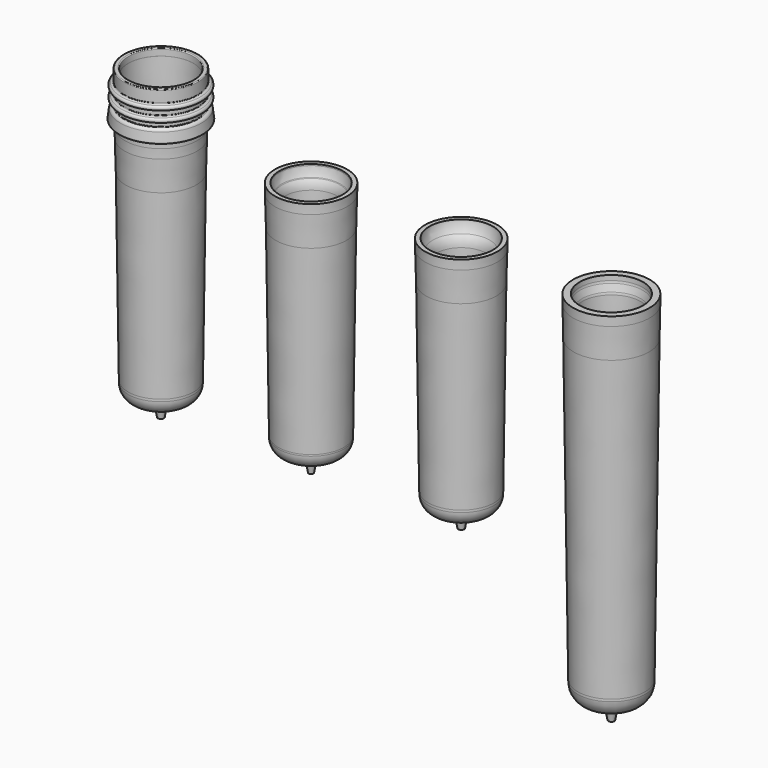
from build123d import *


# Not quite as in the source:
# - ends of sketch curves that miss each other by under 0.0002 mm in the source are joined


with BuildPart() as f2:
    # F1 (on Front) → F2 (revolve)
    with BuildSketch(Plane.XZ):
        with BuildLine():
            Line((-90.380559, 48.017019), (-90.3875184894, 48.4156921852))
            Line((-90.3875184894, 48.4156921852), (-91.848666, 48.396603))
            Line((-91.848666, 48.396603), (-91.808166, 45.296603))
            Line((-91.808166, 45.296603), (-91.546166, 35.296603))
            Line((-91.546166, 35.296603), (-90.748666, -25.603397))
            Line((-90.748666, -25.603397), (-90.724166, -25.603397))
            Line((-90.724166, -25.603397), (-90.714235, -26.362404))
            ThreePointArc((-90.714235, -26.362404), (-89.5797271662, -29.4689449214), (-86.7542219771, -31.1877308925))
            Line((-86.7542219771, -31.1877308925), (-84.798666, -31.603397))
            Line((-84.798666, -31.603397), (-82.5194, -31.603397))
            ThreePointArc((-82.5194, -31.603397), (-81.8766123734, -31.8373525711), (-81.5345922393, -32.4297488659))
            Line((-81.5345922393, -32.4297488659), (-80.798666, -36.603397))
            Line((-80.798666, -36.603397), (-79.797526, -36.603397))
            Line((-79.797526, -36.603397), (-79.797526, -30.103397))
            Line((-79.797526, -30.103397), (-83.797526, -30.103397))
            Line((-83.797526, -30.103397), (-86.010944, -29.163857))
            ThreePointArc((-86.010944, -29.163857), (-87.5492637787, -27.8929535328), (-88.1430844076, -25.9879599922))
            Line((-88.1430844076, -25.9879599922), (-88.945026, 35.296603))
            Line((-88.945026, 35.296603), (-89.032202, 42.663642))
            ThreePointArc((-89.032202, 42.663642), (-89.2114545385, 44.0499692845), (-89.7066271049, 45.3571949455))
            ThreePointArc((-89.7066271049, 45.3571949455), (-90.1976808008, 46.6480650102), (-90.380559, 48.017019))
        make_face()
    revolve(axis=Axis((-79.797526, 0, -33.353397), (0, 0, -1)))


with BuildPart() as f4:
    # F3 (on Front) → F4 (revolve)
    with BuildSketch(Plane.XZ):
        with BuildLine():
            Line((-90.3871852566, 48.396603), (-90.652526, 63.596603))
            Line((-90.652526, 63.596603), (-90.653015, 63.624612))
            Line((-90.653015, 63.624612), (-90.65259, 65.596538))
            ThreePointArc((-90.65259, 65.596538), (-90.7404349859, 65.8087120521), (-90.95259, 65.896603))
            Line((-90.95259, 65.896603), (-91.858666, 65.896603))
            ThreePointArc((-91.858666, 65.896603), (-92.0354426953, 65.8233796953), (-92.108666, 65.646603))
            Line((-92.108666, 65.646603), (-92.108666, 62.896603))
            Line((-92.108666, 62.896603), (-92.108666, 62.036644))
            ThreePointArc((-92.108666, 62.036644), (-92.1448355475, 61.9219287751), (-92.2402618282, 61.8487055279))
            Line((-92.2402618282, 61.8487055279), (-92.962021, 61.586007))
            ThreePointArc((-92.962021, 61.586007), (-93.468666, 60.862443171), (-92.9620211619, 60.1388795552))
            Line((-92.9620211619, 60.1388795552), (-92.240262, 59.876181))
            ThreePointArc((-92.240262, 59.876181), (-92.1448355475, 59.8029582249), (-92.108666, 59.688243))
            Line((-92.108666, 59.688243), (-92.108666, 58.436644))
            ThreePointArc((-92.108666, 58.436644), (-92.1448355475, 58.3219287751), (-92.2402618282, 58.2487055279))
            Line((-92.2402618282, 58.2487055279), (-92.962021, 57.986007))
            ThreePointArc((-92.962021, 57.986007), (-93.468666, 57.262443171), (-92.9620211619, 56.5388795552))
            Line((-92.9620211619, 56.5388795552), (-92.240262, 56.276181))
            ThreePointArc((-92.240262, 56.276181), (-92.1448355475, 56.2029582249), (-92.108666, 56.088243))
            Line((-92.108666, 56.088243), (-92.108666, 55.096597))
            ThreePointArc((-92.108666, 55.096597), (-92.1674728698, 54.9549477854), (-92.3093109999, 54.8965980401))
            ThreePointArc((-92.3093109999, 54.8965980401), (-92.9732916549, 54.6472023083), (-93.3048659973, 54.0202039997))
            Line((-93.3048659973, 54.0202039997), (-93.680325, 51.005841))
            ThreePointArc((-93.680325, 51.005841), (-93.6216260494, 50.7645895992), (-93.4176811572, 50.6229763696))
            Line((-93.4176811572, 50.6229763696), (-92.37932, 50.364085))
            ThreePointArc((-92.37932, 50.364085), (-91.9970582708, 50.1158407746), (-91.848666, 49.684878))
            Line((-91.848666, 49.684878), (-91.848666, 48.396603))
            Line((-91.848666, 48.396603), (-90.3871852566, 48.396603))
        make_face()
    revolve(axis=Axis((-79.798096, 0, -24.73381686), (4.80219e-05, 0, 0.9999999988)))


with BuildPart() as f6:
    # F5 (on Front) → F6 (revolve)
    with BuildSketch(Plane.XZ):
        with BuildLine():
            Line((-41.848666, 48.396603), (-41.808166, 45.296603))
            Line((-41.808166, 45.296603), (-41.546166, 35.296603))
            Line((-41.546166, 35.296603), (-40.748666, -25.603397))
            Line((-40.748666, -25.603397), (-40.742351, -26.085577))
            ThreePointArc((-40.742351, -26.085577), (-39.8806833305, -28.7673156764), (-37.6629290361, -30.5039100939))
            Line((-37.6629290361, -30.5039100939), (-34.798666, -31.603397))
            Line((-34.798666, -31.603397), (-32.3194, -31.603397))
            ThreePointArc((-32.3194, -31.603397), (-31.6766123734, -31.8373525711), (-31.3345922393, -32.4297488659))
            Line((-31.3345922393, -32.4297488659), (-30.598666, -36.603397))
            Line((-30.598666, -36.603397), (-29.798666, -36.603397))
            Line((-29.798666, -36.603397), (-29.798666, -30.003397))
            Line((-29.798666, -30.003397), (-33.798666, -30.003397))
            Line((-33.798666, -30.003397), (-35.5223, -29.271758))
            ThreePointArc((-35.5223, -29.271758), (-37.0606345482, -28.0008325329), (-37.6544411018, -26.0958080013))
            Line((-37.6544411018, -26.0958080013), (-38.458166, 35.296603))
            Line((-38.458166, 35.296603), (-38.533495, 41.673694))
            ThreePointArc((-38.533495, 41.673694), (-38.7601467692, 43.2378397645), (-39.3873628062, 44.6885371162))
            Line((-39.3873628062, 44.6885371162), (-39.526305, 44.920237))
            ThreePointArc((-39.526305, 44.920237), (-40.1488852433, 46.3546530786), (-40.3796770215, 47.9012269996))
            Line((-40.3796770215, 47.9012269996), (-40.3883246154, 48.396603))
            Line((-40.3883246154, 48.396603), (-41.848666, 48.396603))
        make_face()
    revolve(axis=Axis((-29.798666, 0, -12.0286933423), (0, 0, 1)))


with BuildPart() as f8:
    # F7 (on Front) → F8 (revolve)
    with BuildSketch(Plane.XZ):
        with BuildLine():
            Line((9.611341937, 48.4156772972), (8.151334, 48.396603))
            Line((8.151334, 48.396603), (8.191834, 45.296603))
            Line((8.191834, 45.296603), (8.453834, 35.296603))
            Line((8.453834, 35.296603), (9.251334, -25.603397))
            Line((9.251334, -25.603397), (9.275834, -25.603397))
            Line((9.275834, -25.603397), (9.285765, -26.362404))
            ThreePointArc((9.285765, -26.362404), (10.4202728338, -29.4689449214), (13.2457780229, -31.1877308925))
            Line((13.2457780229, -31.1877308925), (15.201334, -31.603397))
            Line((15.201334, -31.603397), (17.4806, -31.603397))
            ThreePointArc((17.4806, -31.603397), (18.1233876266, -31.8373525711), (18.4654077607, -32.4297488659))
            Line((18.4654077607, -32.4297488659), (19.201334, -36.603397))
            Line((19.201334, -36.603397), (20.201334, -36.603397))
            Line((20.201334, -36.603397), (20.201334, -30.003397))
            Line((20.201334, -30.003397), (16.201334, -30.003397))
            Line((16.201334, -30.003397), (14.930215, -29.463839))
            ThreePointArc((14.930215, -29.463839), (13.3918804518, -28.1929135329), (12.7980738982, -26.2878890013))
            Line((12.7980738982, -26.2878890013), (11.991834, 35.296603))
            Line((11.991834, 35.296603), (11.920485, 41.336744))
            ThreePointArc((11.920485, 41.336744), (11.6141133324, 43.1599087139), (10.7672352978, 44.8032562174))
            ThreePointArc((10.7672352978, 44.8032562174), (9.9257232875, 46.4305476153), (9.614479996, 48.235914))
            Line((9.614479996, 48.235914), (9.611341937, 48.4156772972))
        make_face()
    revolve(axis=Axis((20.201334, 0, -33.303397), (0, 0, -1)))


with BuildPart() as f10:
    # F9 (on Front) → F10 (revolve)
    with BuildSketch(Plane.XZ):
        with BuildLine():
            Line((59.6414947748, 48.396603), (57.451334, 48.396603))
            Line((57.451334, 48.396603), (57.477334, 45.396603))
            Line((57.477334, 45.396603), (57.651834, 35.396603))
            Line((57.651834, 35.396603), (58.960834, -64.603397))
            Line((58.960834, -64.603397), (58.970816, -65.365899))
            ThreePointArc((58.970816, -65.365899), (60.3095484526, -69.0315905319), (63.6436310327, -71.0597408461))
            Line((63.6436310327, -71.0597408461), (66.201334, -71.603397))
            Line((66.201334, -71.603397), (67.4806, -71.603397))
            ThreePointArc((67.4806, -71.603397), (68.1233876266, -71.8373525711), (68.4654077607, -72.4297488659))
            Line((68.4654077607, -72.4297488659), (69.201334, -76.603397))
            Line((69.201334, -76.603397), (70.201334, -76.603397))
            Line((70.201334, -76.603397), (70.201334, -70.103397))
            Line((70.201334, -70.103397), (67.201334, -70.103397))
            Line((67.201334, -70.103397), (65.626712, -69.681478))
            ThreePointArc((65.626712, -69.681478), (63.2549639935, -68.1175506721), (62.292735149, -65.4445049964))
            Line((62.292735149, -65.4445049964), (61.674834, -40.103395))
            Line((61.674834, -40.103395), (60.636334, 34.39644))
            Line((60.636334, 34.39644), (60.535049, 42.996148))
            ThreePointArc((60.535049, 42.996148), (60.5040197835, 43.3926127099), (60.4208238262, 43.7814899506))
            Line((60.4208238262, 43.7814899506), (59.784049, 46.020451))
            ThreePointArc((59.784049, 46.020451), (59.7021607108, 46.4004323773), (59.6700897321, 46.787812013))
            Line((59.6700897321, 46.787812013), (59.6414947748, 48.396603))
        make_face()
    revolve(axis=Axis((70.201334, 0, -73.353397), (0, 0, -1)))


solid = Compound([f2.part, f4.part, f6.part, f8.part, f10.part])
